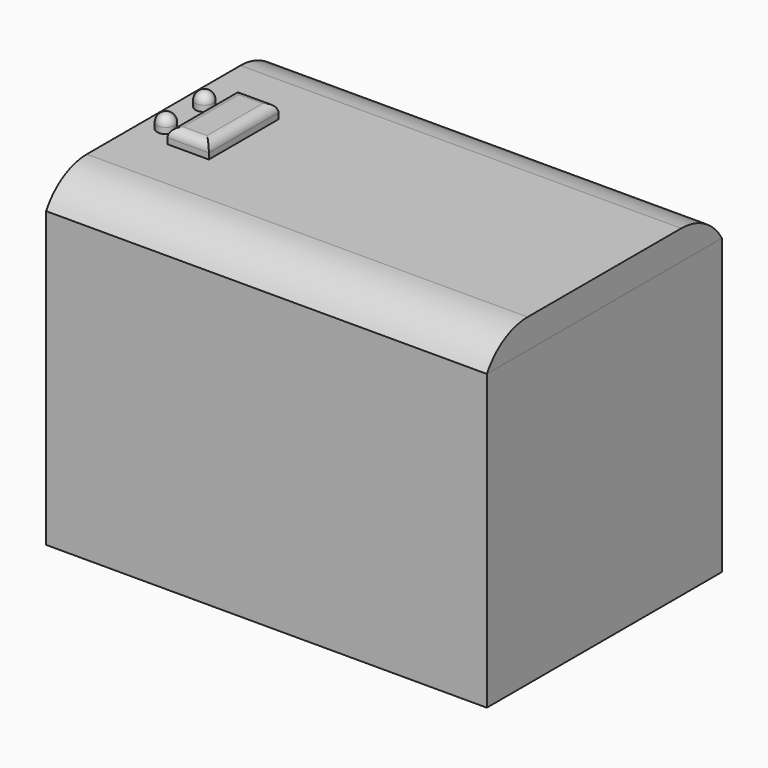
from build123d import *

# Parameters (mm, degrees)
F0_W        = 38.1
F0_H        = 25.4
F1_DEPTH    = 25.4
F0_W_2      = 12.2251660849
F0_H_2      = 22.86
F2_DEPTH    = 2.54
F0_W_3      = 23.3348339151
F0_R        = 7.62
F3_DEPTH    = 2.54
F4_W        = 38.1
F4_H        = 25.4
F5_DEPTH    = 2.54
F6_T1_DEPTH = 44.8570452561
F6_T3_DEPTH = 34.222211341
F7_T1_DEPTH = 60.0970452561
F9_DEPTH    = 6.35
F10_SIZE    = 5.07999
F11_W       = 8.943406865
F11_H       = 17.3965319991
F12_DEPTH   = 12.7
F13_R       = 0.762
F13_W       = 3.5719834268
F13_H       = 7.5215632096
F14_DEPTH   = 2.54
F15_DEPTH   = 1.27
F16_R       = 0.762
F16_2_R     = 0.762
F16_3_R     = 0.762


# Not quite as in the source:
# - a fillet or chamfer that OpenCascade refuses, or shapes differently, is made with other operations: its cross-section is extruded or revolved along the edge and cut away or added
# - a fillet or chamfer is up to 0.001 mm smaller than in the source, because OpenCascade refuses the exact size


with BuildPart() as f1:
    # F0 (on Top) → F1 (new body)
    with BuildSketch(Plane.XY):
        Rectangle(F0_W, F0_H)
        Polygon((-17.78, -11.43), (-17.78, 11.43), (-5.5548339151, 11.43), (17.78, 11.43), (17.78, -11.43), (-5.5548339151, -11.43), align=None, mode=Mode.SUBTRACT)
    extrude(amount=F1_DEPTH)

    # F8 (on face) → F9 (join)
    with BuildSketch(Plane(origin=(-19.05, 0, 0), x_dir=(0, -1, 0), z_dir=(-1, 0, 0))):
        Polygon((-5.08, 0), (0, 0), (5.08, 0), (5.08, 5.08), (0, 5.08), (-5.08, 5.08), align=None)
    extrude(amount=F9_DEPTH)

    # F10 (size 5.08 in the source; OpenCascade refuses exactly that, so slightly less here)
    f10_edges = [f1.edges().sort_by_distance(p)[0] for p in [
        (-25.4, -5.08, 2.54),
        (-25.4, 5.08, 2.54),
    ]]
    chamfer(f10_edges, length=F10_SIZE)


with BuildPart() as f2:
    # F0 (on Top) → F2 (new body)
    with BuildSketch(Plane.XY):
        with Locations((-11.6674169575, 0)):
            Rectangle(F0_W_2, F0_H_2)
    extrude(amount=-F2_DEPTH)

    # F6: fillet of radius 5.08 on 4 edges, made by hand

    # F6_s2 → F6_t1 (cut)
    with BuildSketch(Plane.XZ.offset(-22.4285226281)):
        with BuildLine():
            ThreePointArc((-17.78, 0), (-15.9205909488, -1.8594090512), (-13.3805909488, -2.54))
            Line((-13.3805909488, -2.54), (-17.78, -2.54))
            Line((-17.78, -2.54), (-17.78, 0))
        make_face()
        with BuildLine():
            ThreePointArc((-5.5548339151, 0), (-7.4142429663, -1.8594090512), (-9.9542429663, -2.54))
            Line((-9.9542429663, -2.54), (-5.5548339151, -2.54))
            Line((-5.5548339151, -2.54), (-5.5548339151, 0))
        make_face()
    extrude(amount=F6_T1_DEPTH, mode=Mode.SUBTRACT)

    # F6_s4 → F6_t3 (cut)
    with BuildSketch(Plane.YZ.offset(-28.7785226281)):
        with BuildLine():
            ThreePointArc((-11.43, 0), (-9.5705909488, -1.8594090512), (-7.0305909488, -2.54))
            Line((-7.0305909488, -2.54), (-11.43, -2.54))
            Line((-11.43, -2.54), (-11.43, 0))
        make_face()
        with BuildLine():
            ThreePointArc((11.43, 0), (9.5705909488, -1.8594090512), (7.0305909488, -2.54))
            Line((7.0305909488, -2.54), (11.43, -2.54))
            Line((11.43, -2.54), (11.43, 0))
        make_face()
    extrude(amount=F6_T3_DEPTH, mode=Mode.SUBTRACT)


with BuildPart() as f3:
    # F0 (on Top) → F3 (new body)
    with BuildSketch(Plane.XY):
        with Locations((6.1125830425, 0)):
            Rectangle(F0_W_3, F0_H_2)
        with Locations((6.35, 0)):
            Circle(F0_R, mode=Mode.SUBTRACT)
        with Locations((-11.6674169575, 0)):
            Rectangle(F0_W_2, F0_H_2)
    extrude(amount=F3_DEPTH)


with BuildPart() as f5:
    # F4 (on face) → F5 (new body)
    with BuildSketch(Plane.XY.offset(25.4)):
        Rectangle(F4_W, F4_H)
    extrude(amount=F5_DEPTH)

    # F7: fillet of radius 5.08 on 2 edges, made by hand

    # F7_s2 → F7_t1 (cut)
    with BuildSketch(Plane.YZ.offset(-30.0485226281)):
        with BuildLine():
            ThreePointArc((12.7, 25.4), (10.8405909488, 27.2594090512), (8.3005909488, 27.94))
            Line((8.3005909488, 27.94), (12.7, 27.94))
            Line((12.7, 27.94), (12.7, 25.4))
        make_face()
        with BuildLine():
            ThreePointArc((-12.7, 25.4), (-10.8405909488, 27.2594090512), (-8.3005909488, 27.94))
            Line((-8.3005909488, 27.94), (-12.7, 27.94))
            Line((-12.7, 27.94), (-12.7, 25.4))
        make_face()
    extrude(amount=F7_T1_DEPTH, mode=Mode.SUBTRACT)

    # F13 (on face) → F14 (cut, through all)
    with BuildSketch(Plane.XY.offset(27.94)):
        with Locations((-17.189187929, 2.0751477372)):
            Circle(F13_R)
        with Locations((-17.189187929, -2.0751477372)):
            Circle(F13_R)
        with Locations((-13.9197837561, 0)):
            Rectangle(F13_W, F13_H)
    extrude(amount=-F14_DEPTH, mode=Mode.SUBTRACT)


with BuildPart() as f12:
    # F11 (on face) → F12 (new body)
    with BuildSketch(Plane.XY.offset(2.54)):
        with Locations((-11.2478537485, 0.1831492409)):
            Rectangle(F11_W, F11_H)
    extrude(amount=F12_DEPTH)


with BuildPart() as f15:
    # F13 (on face) → F15 (new body)
    with BuildSketch(Plane.XY.offset(27.94)):
        with Locations((-17.189187929, 2.0751477372)):
            Circle(F13_R)
    extrude(amount=F15_DEPTH)

    # F16
    f16_edges = [f15.edges().sort_by_distance(p)[0] for p in [
        (-17.951188, 2.075148, 29.21),
    ]]
    fillet(f16_edges, radius=F16_R)


with BuildPart() as f15b:
    # F13 (on face) → F15, piece 2 (new body)
    with BuildSketch(Plane.XY.offset(27.94)):
        with Locations((-17.189187929, -2.0751477372)):
            Circle(F13_R)
    extrude(amount=F15_DEPTH)

    # F16#2
    f16_2_edges = [f15b.edges().sort_by_distance(p)[0] for p in [
        (-17.951188, -2.075148, 29.21),
    ]]
    fillet(f16_2_edges, radius=F16_2_R)


with BuildPart() as f15c:
    # F13 (on face) → F15, piece 3 (new body)
    with BuildSketch(Plane.XY.offset(27.94)):
        with Locations((-13.9197837561, 0)):
            Rectangle(F13_W, F13_H)
    extrude(amount=F15_DEPTH)

    # F16#3
    f16_3_edges = [f15c.edges().sort_by_distance(p)[0] for p in [
        (-15.705775, 0, 29.21),
        (-13.919784, -3.760782, 29.21),
        (-12.133792, 0, 29.21),
        (-13.919784, 3.760782, 29.21),
    ]]
    fillet(f16_3_edges, radius=F16_3_R)


solid = Compound([f1.part, f2.part, f3.part, f5.part, f12.part, f15.part, f15b.part, f15c.part])
